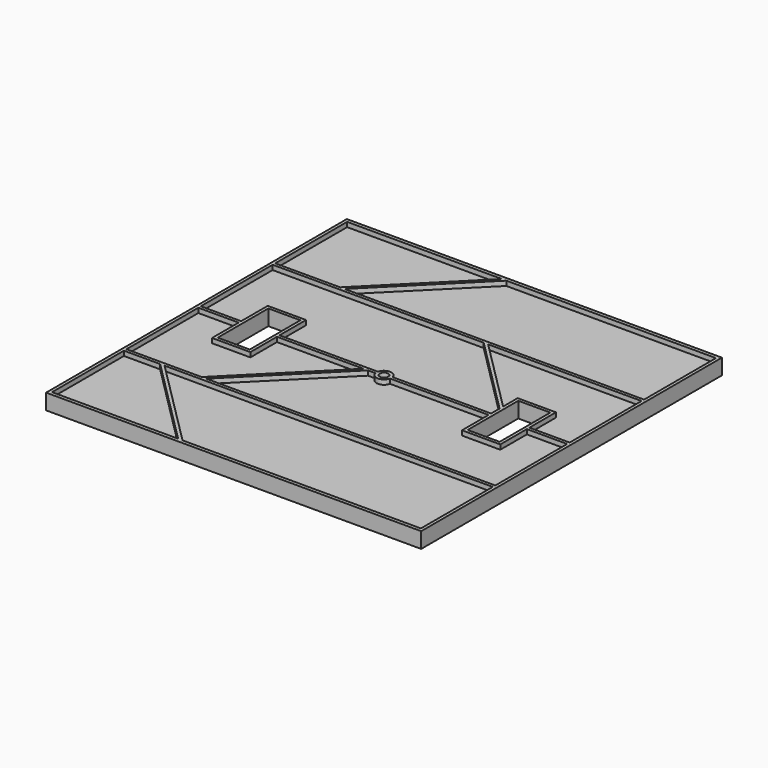
from build123d import *

# Parameters (mm, degrees)
F0_W     = 240.0041820114
F0_H     = 240.5
F0_R     = 2.75
F2_DEPTH = 7
F1_W     = 99.5
F1_H     = 99.5
F3_DEPTH = 7
F4_D     = 5.5
F4_DEPTH = 60
F4_TIP   = 1.6523667023
F5_DEPTH = 10
F7_D     = 6
F7_DEPTH = 2
F7_TIP   = 1.8025818571
F9_D     = 6
F9_DEPTH = 2
F9_TIP   = 1.8025818571


# Not quite as in the source:
# - a feature names something its author has since deleted; it is built from what else it names


with BuildPart() as f2:
    # F0 (on Top) → F2 (new body)
    with BuildSketch(Plane.XY):
        Rectangle(F0_W, F0_H)
        Polygon((-118, -60.5), (-94.8284271247, -60.5), (-37.3284271247, -118), (-118, -118), align=None, mode=Mode.SUBTRACT)
        Polygon((-69.8158430413, -58.5), (-118, -58.5), (-118, -1), (-92.2, -1), (-92.2, -22.25), (-67.7, -22.25), (-67.7, -1), (-12.3158430413, -1), align=None, mode=Mode.SUBTRACT)
        Polygon((118, -118), (-34.5, -118), (-92, -60.5), (118, -60.5), align=None, mode=Mode.SUBTRACT)
        with BuildLine():
            Line((118, -1), (118, -58.5))
            Line((118, -58.5), (-66.9874159165, -58.5))
            Line((-66.9874159165, -58.5), (-9.4874159165, -1))
            Line((-9.4874159165, -1), (-4.6435439053, -1))
            ThreePointArc((-4.6435439053, -1), (0, -4.75), (4.6435439053, -1))
            Line((4.6435439053, -1), (67.6999996539, -1))
            Line((67.6999996539, -1), (67.699995977, -22.25))
            Line((67.699995977, -22.25), (92.2, -22.25))
            Line((92.2, -22.25), (92.2, -1))
            Line((92.2, -1), (118, -1))
        make_face(mode=Mode.SUBTRACT)
        Polygon((-69.7, 20.25), (-69.7, 0), (-69.7, -20.25), (-90.2, -20.25), (-90.2, 0), (-90.2, 20.25), align=None, mode=Mode.SUBTRACT)
        with BuildLine():
            Line((-118.05, 1), (-118.05, 58.5))
            Line((-118.05, 58.5), (16.9895635103, 58.5))
            Line((16.9895635103, 58.5), (67.7, 7.7895635103))
            Line((67.7, 7.7895635103), (67.7, 1))
            Line((67.7, 1), (4.6435439053, 1))
            ThreePointArc((4.6435439053, 1), (0, 4.75), (-4.6435439053, 1))
            Line((-4.6435439053, 1), (-67.7, 1))
            Line((-67.7, 1), (-67.7, 22.25))
            Line((-67.7, 22.25), (-92.2, 22.25))
            Line((-92.2, 22.25), (-92.2, 1))
            Line((-92.2, 1), (-118.05, 1))
        make_face(mode=Mode.SUBTRACT)
        Polygon((-118, 60.5), (-118, 118), (-18.9642378869, 118), (-76.4642378869, 60.5), align=None, mode=Mode.SUBTRACT)
        Circle(F0_R, mode=Mode.SUBTRACT)
        Polygon((69.7, -20.25), (69.7, -2.25), (69.7, 20.25), (90.2, 20.25), (90.2, -2.25), (90.2, -20.25), align=None, mode=Mode.SUBTRACT)
        Polygon((67.7, 22.25), (67.7, 10.617990635), (19.817990635, 58.5), (118, 58.5), (118, 0.9999998737), (92.2, 0.9999998737), (92.2, 22.25), align=None, mode=Mode.SUBTRACT)
        Polygon((118, 118), (118, 60.5), (-73.6358107621, 60.5), (-16.1358107621, 118), align=None, mode=Mode.SUBTRACT)
        Polygon((-92, -60.5), (-34.5, -118), (118, -118), (118, -60.5), align=None)
        Polygon((-73.6358107621, 60.5), (118, 60.5), (118, 118), (-16.1358107621, 118), align=None)
        with BuildLine():
            Line((16.9895635103, 58.5), (-118.05, 58.5))
            Line((-118.05, 58.5), (-118.05, 1))
            Line((-118.05, 1), (-92.2, 1))
            Line((-92.2, 1), (-92.2, 22.25))
            Line((-92.2, 22.25), (-67.7, 22.25))
            Line((-67.7, 22.25), (-67.7, 1))
            Line((-67.7, 1), (-4.6435439053, 1))
            ThreePointArc((-4.6435439053, 1), (0, 4.75), (4.6435439053, 1))
            Line((4.6435439053, 1), (67.7, 1))
            Line((67.7, 1), (67.7, 7.7895635103))
            Line((67.7, 7.7895635103), (16.9895635103, 58.5))
        make_face()
        with BuildLine():
            Line((-66.9874159165, -58.5), (118, -58.5))
            Line((118, -58.5), (118, -1))
            Line((118, -1), (92.2, -1))
            Line((92.2, -1), (92.2, -22.25))
            Line((92.2, -22.25), (67.699995977, -22.25))
            Line((67.699995977, -22.25), (67.6999996539, -1))
            Line((67.6999996539, -1), (4.6435439053, -1))
            ThreePointArc((4.6435439053, -1), (0, -4.75), (-4.6435439053, -1))
            Line((-4.6435439053, -1), (-9.4874159165, -1))
            Line((-9.4874159165, -1), (-66.9874159165, -58.5))
        make_face()
        Polygon((-18.9642378869, 118), (-118, 118), (-118, 60.5), (-76.4642378869, 60.5), align=None)
        Polygon((-118, -1), (-118, -58.5), (-69.8158430413, -58.5), (-12.3158430413, -1), (-67.7, -1), (-67.7, -22.25), (-92.2, -22.25), (-92.2, -1), align=None)
        Polygon((19.817990635, 58.5), (67.7, 10.617990635), (67.7, 22.25), (92.2, 22.25), (92.2, 0.9999998737), (118, 0.9999998737), (118, 58.5), align=None)
        Polygon((-37.3284271247, -118), (-94.8284271247, -60.5), (-118, -60.5), (-118, -118), align=None)
    extrude(amount=F2_DEPTH)

    # F1 (on Top) → F3 (join)
    with BuildSketch(Plane.XY):
        Rectangle(F1_W, F1_H)
    extrude(amount=-F3_DEPTH)

    # F4
    with Locations(Plane.XY):
        with Locations((0, 0)):
            Hole(F4_D / 2, depth=F4_DEPTH)
            with Locations((0, 0, -(F4_DEPTH + F4_TIP / 2))):  # 118° drill point
                Cone(0, F4_D / 2, F4_TIP, mode=Mode.SUBTRACT)

    # F0 (on Top) → F5 (join)
    with BuildSketch(Plane.XY):
        Rectangle(F0_W, F0_H)
        Polygon((-118, -60.5), (-94.8284271247, -60.5), (-37.3284271247, -118), (-118, -118), align=None, mode=Mode.SUBTRACT)
        Polygon((-69.8158430413, -58.5), (-118, -58.5), (-118, -1), (-92.2, -1), (-92.2, -22.25), (-67.7, -22.25), (-67.7, -1), (-12.3158430413, -1), align=None, mode=Mode.SUBTRACT)
        Polygon((118, -118), (-34.5, -118), (-92, -60.5), (118, -60.5), align=None, mode=Mode.SUBTRACT)
        with BuildLine():
            Line((118, -1), (118, -58.5))
            Line((118, -58.5), (-66.9874159165, -58.5))
            Line((-66.9874159165, -58.5), (-9.4874159165, -1))
            Line((-9.4874159165, -1), (-4.6435439053, -1))
            ThreePointArc((-4.6435439053, -1), (0, -4.75), (4.6435439053, -1))
            Line((4.6435439053, -1), (67.6999996539, -1))
            Line((67.6999996539, -1), (67.699995977, -22.25))
            Line((67.699995977, -22.25), (92.2, -22.25))
            Line((92.2, -22.25), (92.2, -1))
            Line((92.2, -1), (118, -1))
        make_face(mode=Mode.SUBTRACT)
        Polygon((-69.7, 20.25), (-69.7, 0), (-69.7, -20.25), (-90.2, -20.25), (-90.2, 0), (-90.2, 20.25), align=None, mode=Mode.SUBTRACT)
        with BuildLine():
            Line((-118.05, 1), (-118.05, 58.5))
            Line((-118.05, 58.5), (16.9895635103, 58.5))
            Line((16.9895635103, 58.5), (67.7, 7.7895635103))
            Line((67.7, 7.7895635103), (67.7, 1))
            Line((67.7, 1), (4.6435439053, 1))
            ThreePointArc((4.6435439053, 1), (0, 4.75), (-4.6435439053, 1))
            Line((-4.6435439053, 1), (-67.7, 1))
            Line((-67.7, 1), (-67.7, 22.25))
            Line((-67.7, 22.25), (-92.2, 22.25))
            Line((-92.2, 22.25), (-92.2, 1))
            Line((-92.2, 1), (-118.05, 1))
        make_face(mode=Mode.SUBTRACT)
        Polygon((-118, 60.5), (-118, 118), (-18.9642378869, 118), (-76.4642378869, 60.5), align=None, mode=Mode.SUBTRACT)
        Circle(F0_R, mode=Mode.SUBTRACT)
        Polygon((69.7, -20.25), (69.7, -2.25), (69.7, 20.25), (90.2, 20.25), (90.2, -2.25), (90.2, -20.25), align=None, mode=Mode.SUBTRACT)
        Polygon((67.7, 22.25), (67.7, 10.617990635), (19.817990635, 58.5), (118, 58.5), (118, 0.9999998737), (92.2, 0.9999998737), (92.2, 22.25), align=None, mode=Mode.SUBTRACT)
        Polygon((118, 118), (118, 60.5), (-73.6358107621, 60.5), (-16.1358107621, 118), align=None, mode=Mode.SUBTRACT)
    extrude(amount=F5_DEPTH)

    # F7
    with Locations(Plane.XZ.offset(49.75)):
        with Locations((0, -3.5)):
            Hole(F7_D / 2, depth=F7_DEPTH)
            with Locations((0, 0, -(F7_DEPTH + F7_TIP / 2))):  # 118° drill point
                Cone(0, F7_D / 2, F7_TIP, mode=Mode.SUBTRACT)

    # F9
    with Locations(Plane(origin=(0, 49.75, 0), x_dir=(-1, 0, 0), z_dir=(0, 1, 0))):
        with Locations((0, -3.5)):
            Hole(F9_D / 2, depth=F9_DEPTH)
            with Locations((0, 0, -(F9_DEPTH + F9_TIP / 2))):  # 118° drill point
                Cone(0, F9_D / 2, F9_TIP, mode=Mode.SUBTRACT)


solid = f2.part
